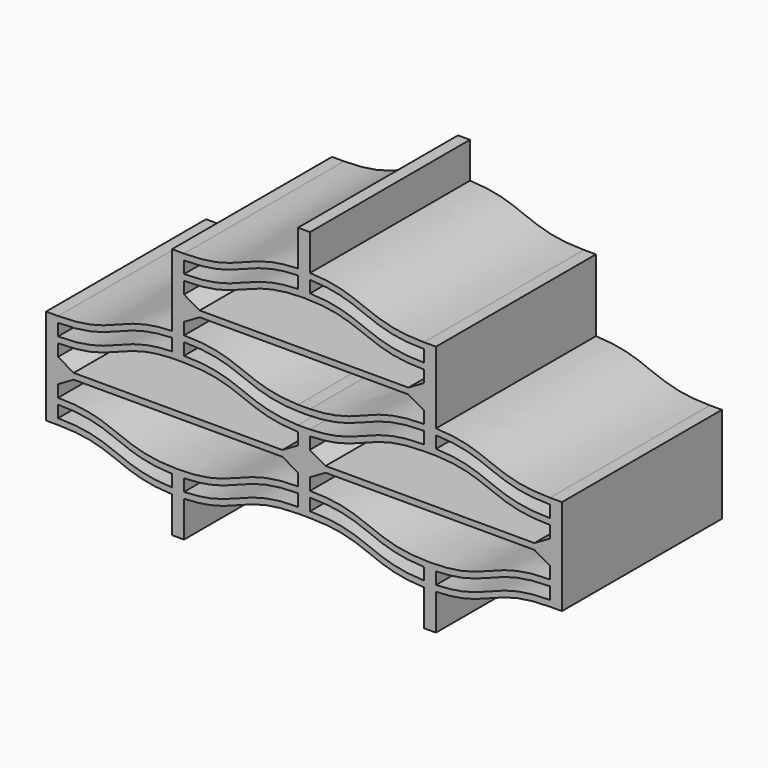
from build123d import *

# Parameters (mm, degrees)
F1_DEPTH = 25


with BuildPart() as f1:
    # F0 (on Front) → F1 (new body)
    with BuildSketch(Plane.XZ):
        with BuildLine():
            Line((1.5, 0), (0, 0))
            Line((0, 0), (0, -12))
            Line((0, -12), (1.5, -12))
            add(Edge.make_bspline(
                [(15.75, -14.9895365677), (12.4912804731, -14.8965121892), (8.8706402366, -13.4482560946), (5.25, -12), (1.5, -12)],
                knots=[0.0344959369, 0.0344959369, 0.0344959369, 0.0344959369, 0.5, 1, 1, 1, 1], degree=3))
            add(Edge.make_bspline(
                [(16.5, -15), (16.2412804731, -15), (15.9914857187, -14.996430091), (15.75, -14.9895365677)],
                knots=[0, 0, 0, 0, 0.0344959369, 0.0344959369, 0.0344959369, 0.0344959369], degree=3))
            add(Edge.make_bspline(
                [(17.25, -14.9895365677), (17.0085142813, -14.996430091), (16.7587195269, -15), (16.5, -15)],
                knots=[0.9655040631, 0.9655040631, 0.9655040631, 0.9655040631, 1, 1, 1, 1], degree=3))
            add(Edge.make_bspline(
                [(31.5, -12), (27.75, -12), (24.1293597634, -13.4482560946), (20.5087195269, -14.8965121892), (17.25, -14.9895365677)],
                knots=[0, 0, 0, 0, 0.5, 0.9655040631, 0.9655040631, 0.9655040631, 0.9655040631], degree=3))
            Line((31.5, -12), (33, -12))
            add(Edge.make_bspline(
                [(47.25, -14.9895365677), (43.9912804731, -14.8965121892), (40.3706402366, -13.4482560946), (36.75, -12), (33, -12)],
                knots=[0.0344959369, 0.0344959369, 0.0344959369, 0.0344959369, 0.5, 1, 1, 1, 1], degree=3))
            add(Edge.make_bspline(
                [(48, -15), (47.7412804731, -15), (47.4914857187, -14.996430091), (47.25, -14.9895365677)],
                knots=[0, 0, 0, 0, 0.0344959369, 0.0344959369, 0.0344959369, 0.0344959369], degree=3))
            add(Edge.make_bspline(
                [(48.75, -14.9895365677), (48.5085142813, -14.996430091), (48.2587195269, -15), (48, -15)],
                knots=[0.9655040631, 0.9655040631, 0.9655040631, 0.9655040631, 1, 1, 1, 1], degree=3))
            add(Edge.make_bspline(
                [(63, -12), (59.25, -12), (55.6293597634, -13.4482560946), (52.0087195269, -14.8965121892), (48.75, -14.9895365677)],
                knots=[0, 0, 0, 0, 0.5, 0.9655040631, 0.9655040631, 0.9655040631, 0.9655040631], degree=3))
            Line((63, -12), (64.5, -12))
            Line((64.5, -12), (64.5, 0))
            Line((64.5, 0), (63, 0))
            add(Edge.make_bspline(
                [(48.75, 2.9895365677), (52.0087195269, 2.8965121892), (55.6293597634, 1.4482560946), (59.25, 0), (63, 0)],
                knots=[0.0344959369, 0.0344959369, 0.0344959369, 0.0344959369, 0.5, 1, 1, 1, 1], degree=3))
            Line((48.75, 2.9895365677), (48.75, 7.4895365677))
            Line((48.75, 7.4895365677), (48.75, 11.9895365677))
            Line((48.75, 11.9895365677), (47.25, 11.9895365677))
            add(Edge.make_bspline(
                [(33, 14.9790731355), (36.2587195269, 14.886048757), (39.8793597634, 13.4377926624), (43.5, 11.9895365677), (47.25, 11.9895365677)],
                knots=[0.0344959369, 0.0344959369, 0.0344959369, 0.0344959369, 0.5, 1, 1, 1, 1], degree=3))
            add(Edge.make_bspline(
                [(32.25, 14.9895365677), (32.5087195269, 14.9895365677), (32.7585142813, 14.9859666587), (33, 14.9790731355)],
                knots=[0, 0, 0, 0, 0.0344959369, 0.0344959369, 0.0344959369, 0.0344959369], degree=3))
            add(Edge.make_bspline(
                [(31.5, 14.9790731355), (31.7414857187, 14.9859666587), (31.9912804731, 14.9895365677), (32.25, 14.9895365677)],
                knots=[0.9655040631, 0.9655040631, 0.9655040631, 0.9655040631, 1, 1, 1, 1], degree=3))
            add(Edge.make_bspline(
                [(17.25, 11.9895365677), (21, 11.9895365677), (24.6206402366, 13.4377926624), (28.2412804731, 14.886048757), (31.5, 14.9790731355)],
                knots=[0, 0, 0, 0, 0.5, 0.9655040631, 0.9655040631, 0.9655040631, 0.9655040631], degree=3))
            Line((17.25, 11.9895365677), (15.75, 11.9895365677))
            Line((15.75, 11.9895365677), (15.75, 7.4895365677))
            Line((15.75, 7.4895365677), (15.75, 2.9895365677))
            add(Edge.make_bspline(
                [(1.5, 0), (5.25, 0), (8.8706402366, 1.4482560946), (12.4912804731, 2.8965121892), (15.75, 2.9895365677)],
                knots=[0, 0, 0, 0, 0.5, 0.9655040631, 0.9655040631, 0.9655040631, 0.9655040631], degree=3))
        make_face()
        with BuildLine():
            Line((1.5, -11.25), (1.5, -9.75))
            add(Edge.make_bspline(
                [(15.75, -12.7395365677), (12.4912804731, -12.6465121892), (8.8706402366, -11.1982560946), (5.25, -9.75), (1.5, -9.75)],
                knots=[0.0344959369, 0.0344959369, 0.0344959369, 0.0344959369, 0.5, 1, 1, 1, 1], degree=3))
            add(Edge.make_bspline(
                [(16.5, -12.75), (16.2412804731, -12.75), (15.9914857187, -12.746430091), (15.75, -12.7395365677)],
                knots=[0, 0, 0, 0, 0.0344959369, 0.0344959369, 0.0344959369, 0.0344959369], degree=3))
            add(Edge.make_bspline(
                [(17.25, -12.7395365677), (17.0085142813, -12.746430091), (16.7587195269, -12.75), (16.5, -12.75)],
                knots=[0.9655040631, 0.9655040631, 0.9655040631, 0.9655040631, 1, 1, 1, 1], degree=3))
            add(Edge.make_bspline(
                [(31.5, -9.75), (27.75, -9.75), (24.1293597634, -11.1982560946), (20.5087195269, -12.6465121892), (17.25, -12.7395365677)],
                knots=[0, 0, 0, 0, 0.5, 0.9655040631, 0.9655040631, 0.9655040631, 0.9655040631], degree=3))
            Line((31.5, -9.75), (31.5, -11.25))
            add(Edge.make_bspline(
                [(31.5, -11.25), (27.75, -11.25), (24.1293597634, -12.6982560946), (20.5087195269, -14.1465121892), (17.25, -14.2395365677)],
                knots=[0, 0, 0, 0, 0.5, 0.9655040631, 0.9655040631, 0.9655040631, 0.9655040631], degree=3))
            add(Edge.make_bspline(
                [(17.25, -14.2395365677), (17.0085142813, -14.246430091), (16.7587195269, -14.25), (16.5, -14.25)],
                knots=[0.9655040631, 0.9655040631, 0.9655040631, 0.9655040631, 1, 1, 1, 1], degree=3))
            add(Edge.make_bspline(
                [(16.5, -14.25), (16.2412804731, -14.25), (15.9914857187, -14.246430091), (15.75, -14.2395365677)],
                knots=[0, 0, 0, 0, 0.0344959369, 0.0344959369, 0.0344959369, 0.0344959369], degree=3))
            add(Edge.make_bspline(
                [(15.75, -14.2395365677), (12.4912804731, -14.1465121892), (8.8706402366, -12.6982560946), (5.25, -11.25), (1.5, -11.25)],
                knots=[0.0344959369, 0.0344959369, 0.0344959369, 0.0344959369, 0.5, 1, 1, 1, 1], degree=3))
        make_face(mode=Mode.SUBTRACT)
        with BuildLine():
            Line((1.5, -2.25), (1.5, -0.75))
            add(Edge.make_bspline(
                [(1.5, -0.75), (5.25, -0.75), (8.8706402366, 0.6982560946), (12.4912804731, 2.1465121892), (15.75, 2.2395365677)],
                knots=[0, 0, 0, 0, 0.5, 0.9655040631, 0.9655040631, 0.9655040631, 0.9655040631], degree=3))
            Line((15.75, 2.2395365677), (15.75, 0.7395365677))
            add(Edge.make_bspline(
                [(1.5, -2.25), (5.25, -2.25), (8.8706402366, -0.8017439054), (12.4912804731, 0.6465121892), (15.75, 0.7395365677)],
                knots=[0, 0, 0, 0, 0.5, 0.9655040631, 0.9655040631, 0.9655040631, 0.9655040631], degree=3))
        make_face(mode=Mode.SUBTRACT)
        with BuildLine():
            Line((1.5, -9), (1.5, -7.5))
            Line((1.5, -7.5), (3.4485571585, -6.375))
            Line((3.4485571585, -6.375), (29.5514428415, -6.375))
            Line((29.5514428415, -6.375), (31.5, -7.5))
            Line((31.5, -7.5), (31.5, -9))
            add(Edge.make_bspline(
                [(31.5, -9), (27.75, -9), (24, -10.5), (20.25, -12), (16.5, -12)],
                knots=[0, 0, 0, 0, 0.5, 1, 1, 1, 1], degree=3))
            add(Edge.make_bspline(
                [(16.5, -12), (12.75, -12), (9, -10.5), (5.25, -9), (1.5, -9)],
                knots=[0, 0, 0, 0, 0.5, 1, 1, 1, 1], degree=3))
        make_face(mode=Mode.SUBTRACT)
        with BuildLine():
            Line((3.4485571585, -5.625), (1.5, -4.5))
            Line((1.5, -4.5), (1.5, -3))
            add(Edge.make_bspline(
                [(1.5, -3), (5.25, -3), (8.8706402366, -1.5517439054), (12.4912804731, -0.1034878108), (15.75, -0.0104634323)],
                knots=[0, 0, 0, 0, 0.5, 0.9655040631, 0.9655040631, 0.9655040631, 0.9655040631], degree=3))
            add(Edge.make_bspline(
                [(15.75, -0.0104634323), (15.9914857187, -0.003569909), (16.2412804731, 0), (16.5, 0)],
                knots=[0.9655040631, 0.9655040631, 0.9655040631, 0.9655040631, 1, 1, 1, 1], degree=3))
            add(Edge.make_bspline(
                [(16.5, 0), (16.7587195269, 0), (17.0085142813, -0.003569909), (17.25, -0.0104634323)],
                knots=[0, 0, 0, 0, 0.0344959369, 0.0344959369, 0.0344959369, 0.0344959369], degree=3))
            add(Edge.make_bspline(
                [(31.5, -3), (28.2412804731, -2.9069756215), (24.6206402366, -1.4587195269), (21, -0.0104634323), (17.25, -0.0104634323)],
                knots=[0.0344959369, 0.0344959369, 0.0344959369, 0.0344959369, 0.5, 1, 1, 1, 1], degree=3))
            Line((31.5, -3), (31.5, -4.5))
            Line((31.5, -4.5), (29.5514428415, -5.625))
            Line((29.5514428415, -5.625), (16.5, -5.625))
            Line((16.5, -5.625), (3.4485571585, -5.625))
        make_face(mode=Mode.SUBTRACT)
        with BuildLine():
            Line((33, -11.25), (33, -9.75))
            add(Edge.make_bspline(
                [(47.25, -12.7395365677), (43.9912804731, -12.6465121892), (40.3706402366, -11.1982560946), (36.75, -9.75), (33, -9.75)],
                knots=[0.0344959369, 0.0344959369, 0.0344959369, 0.0344959369, 0.5, 1, 1, 1, 1], degree=3))
            add(Edge.make_bspline(
                [(48, -12.75), (47.7412804731, -12.75), (47.4914857187, -12.746430091), (47.25, -12.7395365677)],
                knots=[0, 0, 0, 0, 0.0344959369, 0.0344959369, 0.0344959369, 0.0344959369], degree=3))
            add(Edge.make_bspline(
                [(48.75, -12.7395365677), (48.5085142813, -12.746430091), (48.2587195269, -12.75), (48, -12.75)],
                knots=[0.9655040631, 0.9655040631, 0.9655040631, 0.9655040631, 1, 1, 1, 1], degree=3))
            add(Edge.make_bspline(
                [(63, -9.75), (59.25, -9.75), (55.6293597634, -11.1982560946), (52.0087195269, -12.6465121892), (48.75, -12.7395365677)],
                knots=[0, 0, 0, 0, 0.5, 0.9655040631, 0.9655040631, 0.9655040631, 0.9655040631], degree=3))
            Line((63, -9.75), (63, -11.25))
            add(Edge.make_bspline(
                [(63, -11.25), (59.25, -11.25), (55.6293597634, -12.6982560946), (52.0087195269, -14.1465121892), (48.75, -14.2395365677)],
                knots=[0, 0, 0, 0, 0.5, 0.9655040631, 0.9655040631, 0.9655040631, 0.9655040631], degree=3))
            add(Edge.make_bspline(
                [(48.75, -14.2395365677), (48.5085142813, -14.246430091), (48.2587195269, -14.25), (48, -14.25)],
                knots=[0.9655040631, 0.9655040631, 0.9655040631, 0.9655040631, 1, 1, 1, 1], degree=3))
            add(Edge.make_bspline(
                [(48, -14.25), (47.7412804731, -14.25), (47.4914857187, -14.246430091), (47.25, -14.2395365677)],
                knots=[0, 0, 0, 0, 0.0344959369, 0.0344959369, 0.0344959369, 0.0344959369], degree=3))
            add(Edge.make_bspline(
                [(47.25, -14.2395365677), (43.9912804731, -14.1465121892), (40.3706402366, -12.6982560946), (36.75, -11.25), (33, -11.25)],
                knots=[0.0344959369, 0.0344959369, 0.0344959369, 0.0344959369, 0.5, 1, 1, 1, 1], degree=3))
        make_face(mode=Mode.SUBTRACT)
        with BuildLine():
            Line((33, -9), (33, -7.5))
            Line((33, -7.5), (34.9485571585, -6.375))
            Line((34.9485571585, -6.375), (61.0514428415, -6.375))
            Line((61.0514428415, -6.375), (63, -7.5))
            Line((63, -7.5), (63, -9))
            add(Edge.make_bspline(
                [(63, -9), (59.25, -9), (55.5, -10.5), (51.75, -12), (48, -12)],
                knots=[0, 0, 0, 0, 0.5, 1, 1, 1, 1], degree=3))
            add(Edge.make_bspline(
                [(48, -12), (44.25, -12), (40.5, -10.5), (36.75, -9), (33, -9)],
                knots=[0, 0, 0, 0, 0.5, 1, 1, 1, 1], degree=3))
        make_face(mode=Mode.SUBTRACT)
        with BuildLine():
            Line((17.25, 0.7395365677), (17.25, 2.2395365677))
            add(Edge.make_bspline(
                [(32.25, -0.7604634323), (28.5, -0.7604634323), (24.75, 0.7395365677), (21, 2.2395365677), (17.25, 2.2395365677)],
                knots=[0, 0, 0, 0, 0.5, 1, 1, 1, 1], degree=3))
            add(Edge.make_bspline(
                [(47.25, 2.2395365677), (43.5, 2.2395365677), (39.75, 0.7395365677), (36, -0.7604634323), (32.25, -0.7604634323)],
                knots=[0, 0, 0, 0, 0.5, 1, 1, 1, 1], degree=3))
            Line((47.25, 2.2395365677), (47.25, 0.7395365677))
            add(Edge.make_bspline(
                [(47.25, 0.7395365677), (43.5, 0.7395365677), (39.8746812443, -0.7105909346), (36.2493624885, -2.1607184368), (32.9737661217, -2.2507348947)],
                knots=[0, 0, 0, 0, 0.5, 0.9667516682, 0.9667516682, 0.9667516682, 0.9667516682], degree=3))
            add(Edge.make_bspline(
                [(32.9737661217, -2.2507348947), (32.7404340903, -2.2571470776), (32.4993624885, -2.2604634323), (32.25, -2.2604634323)],
                knots=[0.9667516682, 0.9667516682, 0.9667516682, 0.9667516682, 1, 1, 1, 1], degree=3))
            add(Edge.make_bspline(
                [(32.25, -2.2604634323), (31.9912804731, -2.2604634323), (31.7414857187, -2.2568935233), (31.5, -2.25)],
                knots=[0, 0, 0, 0, 0.0344959369, 0.0344959369, 0.0344959369, 0.0344959369], degree=3))
            add(Edge.make_bspline(
                [(31.5, -2.25), (28.2412804731, -2.1569756215), (24.6206402366, -0.7087195269), (21, 0.7395365677), (17.25, 0.7395365677)],
                knots=[0.0344959369, 0.0344959369, 0.0344959369, 0.0344959369, 0.5, 1, 1, 1, 1], degree=3))
        make_face(mode=Mode.SUBTRACT)
        with BuildLine():
            Line((32.9737661217, -4.5), (32.9737661217, -3.0007348947))
            add(Edge.make_bspline(
                [(47.25, -0.0104634323), (43.5, -0.0104634323), (39.8746812443, -1.4605909346), (36.2493624885, -2.9107184368), (32.9737661217, -3.0007348947)],
                knots=[0, 0, 0, 0, 0.5, 0.9667516682, 0.9667516682, 0.9667516682, 0.9667516682], degree=3))
            Line((47.25, -0.0104634323), (48.75, -0.0104634323))
            add(Edge.make_bspline(
                [(48.75, -0.0104634323), (52.0087195269, -0.1034878108), (55.6293597634, -1.5517439054), (59.25, -3), (63, -3)],
                knots=[0.0344959369, 0.0344959369, 0.0344959369, 0.0344959369, 0.5, 1, 1, 1, 1], degree=3))
            Line((63, -3), (63, -4.5))
            Line((63, -4.5), (61.0514428415, -5.625))
            Line((61.0514428415, -5.625), (48, -5.625))
            Line((48, -5.625), (34.9485571585, -5.625))
            Line((34.9485571585, -5.625), (32.9737661217, -4.5))
        make_face(mode=Mode.SUBTRACT)
        with BuildLine():
            add(Edge.make_bspline(
                [(48.75, 2.2395365677), (52.0087195269, 2.1465121892), (55.6293597634, 0.6982560946), (59.25, -0.75), (63, -0.75)],
                knots=[0.0344959369, 0.0344959369, 0.0344959369, 0.0344959369, 0.5, 1, 1, 1, 1], degree=3))
            Line((63, -0.75), (63, -2.25))
            add(Edge.make_bspline(
                [(48.75, 0.7395365677), (52.0087195269, 0.6465121892), (55.6293597634, -0.8017439054), (59.25, -2.25), (63, -2.25)],
                knots=[0.0344959369, 0.0344959369, 0.0344959369, 0.0344959369, 0.5, 1, 1, 1, 1], degree=3))
            Line((48.75, 0.7395365677), (48.75, 2.2395365677))
        make_face(mode=Mode.SUBTRACT)
        with BuildLine():
            add(Edge.make_bspline(
                [(47.25, 2.9895365677), (43.5, 2.9895365677), (39.8793597634, 1.5412804731), (36.2587195269, 0.0930243785), (33, 0)],
                knots=[0, 0, 0, 0, 0.5, 0.9655040631, 0.9655040631, 0.9655040631, 0.9655040631], degree=3))
            add(Edge.make_bspline(
                [(33, 0), (32.7585142813, -0.0068935233), (32.5087195269, -0.0104634323), (32.25, -0.0104634323)],
                knots=[0.9655040631, 0.9655040631, 0.9655040631, 0.9655040631, 1, 1, 1, 1], degree=3))
            add(Edge.make_bspline(
                [(32.25, -0.0104634323), (31.9912804731, -0.0104634323), (31.7414857187, -0.0068935233), (31.5, 0)],
                knots=[0, 0, 0, 0, 0.0344959369, 0.0344959369, 0.0344959369, 0.0344959369], degree=3))
            add(Edge.make_bspline(
                [(31.5, 0), (28.2412804731, 0.0930243785), (24.6206402366, 1.5412804731), (21, 2.9895365677), (17.25, 2.9895365677)],
                knots=[0.0344959369, 0.0344959369, 0.0344959369, 0.0344959369, 0.5, 1, 1, 1, 1], degree=3))
            Line((17.25, 2.9895365677), (17.25, 4.4895365677))
            Line((17.25, 4.4895365677), (19.1985571585, 5.6145365677))
            Line((19.1985571585, 5.6145365677), (45.3014428415, 5.6145365677))
            Line((45.3014428415, 5.6145365677), (47.25, 4.4895365677))
            Line((47.25, 4.4895365677), (47.25, 2.9895365677))
        make_face(mode=Mode.SUBTRACT)
        with BuildLine():
            Line((19.1985571585, 6.3645365677), (17.25, 7.4895365677))
            Line((17.25, 7.4895365677), (17.25, 8.9895365677))
            add(Edge.make_bspline(
                [(17.25, 8.9895365677), (21, 8.9895365677), (24.75, 10.4895365677), (28.5, 11.9895365677), (32.25, 11.9895365677)],
                knots=[0, 0, 0, 0, 0.5, 1, 1, 1, 1], degree=3))
            add(Edge.make_bspline(
                [(32.25, 11.9895365677), (36, 11.9895365677), (39.75, 10.4895365677), (43.5, 8.9895365677), (47.25, 8.9895365677)],
                knots=[0, 0, 0, 0, 0.5, 1, 1, 1, 1], degree=3))
            Line((47.25, 8.9895365677), (47.25, 7.4895365677))
            Line((47.25, 7.4895365677), (45.3014428415, 6.3645365677))
            Line((45.3014428415, 6.3645365677), (32.25, 6.3645365677))
            Line((32.25, 6.3645365677), (19.1985571585, 6.3645365677))
        make_face(mode=Mode.SUBTRACT)
        with BuildLine():
            Line((17.25, 9.7395365677), (17.25, 11.2395365677))
            add(Edge.make_bspline(
                [(17.25, 11.2395365677), (21, 11.2395365677), (24.6206402366, 12.6877926624), (28.2412804731, 14.136048757), (31.5, 14.2290731355)],
                knots=[0, 0, 0, 0, 0.5, 0.9655040631, 0.9655040631, 0.9655040631, 0.9655040631], degree=3))
            add(Edge.make_bspline(
                [(31.5, 14.2290731355), (31.7414857187, 14.2359666587), (31.9912804731, 14.2395365677), (32.25, 14.2395365677)],
                knots=[0.9655040631, 0.9655040631, 0.9655040631, 0.9655040631, 1, 1, 1, 1], degree=3))
            add(Edge.make_bspline(
                [(32.25, 14.2395365677), (32.5087195269, 14.2395365677), (32.7585142813, 14.2359666587), (33, 14.2290731355)],
                knots=[0, 0, 0, 0, 0.0344959369, 0.0344959369, 0.0344959369, 0.0344959369], degree=3))
            add(Edge.make_bspline(
                [(33, 14.2290731355), (36.2587195269, 14.136048757), (39.8793597634, 12.6877926624), (43.5, 11.2395365677), (47.25, 11.2395365677)],
                knots=[0.0344959369, 0.0344959369, 0.0344959369, 0.0344959369, 0.5, 1, 1, 1, 1], degree=3))
            Line((47.25, 11.2395365677), (47.25, 9.7395365677))
            add(Edge.make_bspline(
                [(33, 12.7290731355), (36.2587195269, 12.636048757), (39.8793597634, 11.1877926624), (43.5, 9.7395365677), (47.25, 9.7395365677)],
                knots=[0.0344959369, 0.0344959369, 0.0344959369, 0.0344959369, 0.5, 1, 1, 1, 1], degree=3))
            add(Edge.make_bspline(
                [(32.25, 12.7395365677), (32.5087195269, 12.7395365677), (32.7585142813, 12.7359666587), (33, 12.7290731355)],
                knots=[0, 0, 0, 0, 0.0344959369, 0.0344959369, 0.0344959369, 0.0344959369], degree=3))
            add(Edge.make_bspline(
                [(31.5, 12.7290731355), (31.7414857187, 12.7359666587), (31.9912804731, 12.7395365677), (32.25, 12.7395365677)],
                knots=[0.9655040631, 0.9655040631, 0.9655040631, 0.9655040631, 1, 1, 1, 1], degree=3))
            add(Edge.make_bspline(
                [(17.25, 9.7395365677), (21, 9.7395365677), (24.6206402366, 11.1877926624), (28.2412804731, 12.636048757), (31.5, 12.7290731355)],
                knots=[0, 0, 0, 0, 0.5, 0.9655040631, 0.9655040631, 0.9655040631, 0.9655040631], degree=3))
        make_face(mode=Mode.SUBTRACT)
        with BuildLine():
            add(Edge.make_bspline(
                [(16.5, -15), (16.2412804731, -15), (15.9914857187, -14.996430091), (15.75, -14.9895365677)],
                knots=[0, 0, 0, 0, 0.0344959369, 0.0344959369, 0.0344959369, 0.0344959369], degree=3))
            Line((15.75, -14.9895365677), (15.75, -19.4895365677))
            Line((15.75, -19.4895365677), (17.25, -19.4895365677))
            Line((17.25, -19.4895365677), (17.25, -14.9895365677))
            add(Edge.make_bspline(
                [(17.25, -14.9895365677), (17.0085142813, -14.996430091), (16.7587195269, -15), (16.5, -15)],
                knots=[0.9655040631, 0.9655040631, 0.9655040631, 0.9655040631, 1, 1, 1, 1], degree=3))
        make_face()
        with BuildLine():
            Line((31.5, 19.4790731355), (31.5, 14.9790731355))
            add(Edge.make_bspline(
                [(31.5, 14.9790731355), (31.7414857187, 14.9859666587), (31.9912804731, 14.9895365677), (32.25, 14.9895365677)],
                knots=[0.9655040631, 0.9655040631, 0.9655040631, 0.9655040631, 1, 1, 1, 1], degree=3))
            add(Edge.make_bspline(
                [(32.25, 14.9895365677), (32.5087195269, 14.9895365677), (32.7585142813, 14.9859666587), (33, 14.9790731355)],
                knots=[0, 0, 0, 0, 0.0344959369, 0.0344959369, 0.0344959369, 0.0344959369], degree=3))
            Line((33, 14.9790731355), (33, 19.4790731355))
            Line((33, 19.4790731355), (31.5, 19.4790731355))
        make_face()
        with BuildLine():
            add(Edge.make_bspline(
                [(48, -15), (47.7412804731, -15), (47.4914857187, -14.996430091), (47.25, -14.9895365677)],
                knots=[0, 0, 0, 0, 0.0344959369, 0.0344959369, 0.0344959369, 0.0344959369], degree=3))
            Line((47.25, -14.9895365677), (47.25, -19.4895365677))
            Line((47.25, -19.4895365677), (48.75, -19.4895365677))
            Line((48.75, -19.4895365677), (48.75, -14.9895365677))
            add(Edge.make_bspline(
                [(48.75, -14.9895365677), (48.5085142813, -14.996430091), (48.2587195269, -15), (48, -15)],
                knots=[0.9655040631, 0.9655040631, 0.9655040631, 0.9655040631, 1, 1, 1, 1], degree=3))
        make_face()
        with BuildLine():
            add(Edge.make_bspline(
                [(16.5, -12.75), (16.2412804731, -12.75), (15.9914857187, -12.746430091), (15.75, -12.7395365677)],
                knots=[0, 0, 0, 0, 0.0344959369, 0.0344959369, 0.0344959369, 0.0344959369], degree=3))
            Line((15.75, -12.7395365677), (15.75, -14.2395365677))
            add(Edge.make_bspline(
                [(16.5, -14.25), (16.2412804731, -14.25), (15.9914857187, -14.246430091), (15.75, -14.2395365677)],
                knots=[0, 0, 0, 0, 0.0344959369, 0.0344959369, 0.0344959369, 0.0344959369], degree=3))
            add(Edge.make_bspline(
                [(17.25, -14.2395365677), (17.0085142813, -14.246430091), (16.7587195269, -14.25), (16.5, -14.25)],
                knots=[0.9655040631, 0.9655040631, 0.9655040631, 0.9655040631, 1, 1, 1, 1], degree=3))
            Line((17.25, -14.2395365677), (17.25, -12.7395365677))
            add(Edge.make_bspline(
                [(17.25, -12.7395365677), (17.0085142813, -12.746430091), (16.7587195269, -12.75), (16.5, -12.75)],
                knots=[0.9655040631, 0.9655040631, 0.9655040631, 0.9655040631, 1, 1, 1, 1], degree=3))
        make_face()
        with BuildLine():
            add(Edge.make_bspline(
                [(48, -12.75), (47.7412804731, -12.75), (47.4914857187, -12.746430091), (47.25, -12.7395365677)],
                knots=[0, 0, 0, 0, 0.0344959369, 0.0344959369, 0.0344959369, 0.0344959369], degree=3))
            Line((47.25, -12.7395365677), (47.25, -14.2395365677))
            add(Edge.make_bspline(
                [(48, -14.25), (47.7412804731, -14.25), (47.4914857187, -14.246430091), (47.25, -14.2395365677)],
                knots=[0, 0, 0, 0, 0.0344959369, 0.0344959369, 0.0344959369, 0.0344959369], degree=3))
            add(Edge.make_bspline(
                [(48.75, -14.2395365677), (48.5085142813, -14.246430091), (48.2587195269, -14.25), (48, -14.25)],
                knots=[0.9655040631, 0.9655040631, 0.9655040631, 0.9655040631, 1, 1, 1, 1], degree=3))
            Line((48.75, -14.2395365677), (48.75, -12.7395365677))
            add(Edge.make_bspline(
                [(48.75, -12.7395365677), (48.5085142813, -12.746430091), (48.2587195269, -12.75), (48, -12.75)],
                knots=[0.9655040631, 0.9655040631, 0.9655040631, 0.9655040631, 1, 1, 1, 1], degree=3))
        make_face()
        with BuildLine():
            add(Edge.make_bspline(
                [(31.5, 14.2290731355), (31.7414857187, 14.2359666587), (31.9912804731, 14.2395365677), (32.25, 14.2395365677)],
                knots=[0.9655040631, 0.9655040631, 0.9655040631, 0.9655040631, 1, 1, 1, 1], degree=3))
            Line((31.5, 14.2290731355), (31.5, 12.7290731355))
            add(Edge.make_bspline(
                [(31.5, 12.7290731355), (31.7414857187, 12.7359666587), (31.9912804731, 12.7395365677), (32.25, 12.7395365677)],
                knots=[0.9655040631, 0.9655040631, 0.9655040631, 0.9655040631, 1, 1, 1, 1], degree=3))
            add(Edge.make_bspline(
                [(32.25, 12.7395365677), (32.5087195269, 12.7395365677), (32.7585142813, 12.7359666587), (33, 12.7290731355)],
                knots=[0, 0, 0, 0, 0.0344959369, 0.0344959369, 0.0344959369, 0.0344959369], degree=3))
            Line((33, 12.7290731355), (33, 14.2290731355))
            add(Edge.make_bspline(
                [(32.25, 14.2395365677), (32.5087195269, 14.2395365677), (32.7585142813, 14.2359666587), (33, 14.2290731355)],
                knots=[0, 0, 0, 0, 0.0344959369, 0.0344959369, 0.0344959369, 0.0344959369], degree=3))
        make_face()
    extrude(amount=F1_DEPTH)


solid = f1.part
